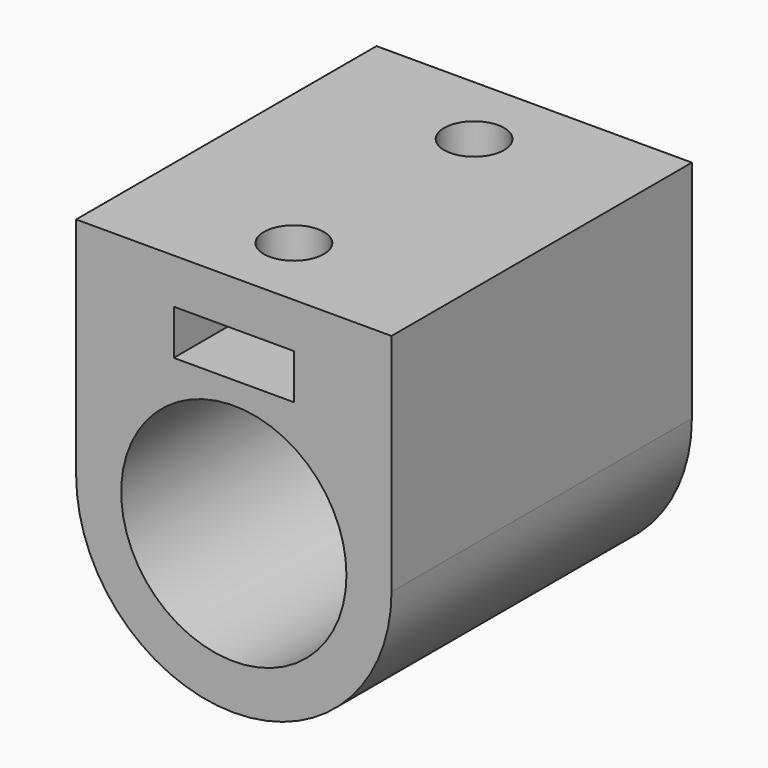
from build123d import *

# Parameters (mm, degrees)
F1_DEPTH        = 25
F2_R            = 2
F3_DEPTH        = 6
F4_W            = 8
F4_H            = 3
F5_DEPTH        = 8
F5_COPIES_COUNT = 2
F5_COPIES_PITCH = 17


# Not quite as in the source:
# - a pattern or mirror of a feature is missing from the dataset's text; its kind, count and spacing are read off the source's solid


with BuildPart() as f1:
    # F0 (on Front) → F1 (new body)
    with BuildSketch(Plane.XZ):
        with BuildLine():
            ThreePointArc((-10.5, 0), (0, 10.5), (10.5, 0))
            Line((10.5, 0), (10.5, 15))
            Line((10.5, 15), (-10.5, 15))
            Line((-10.5, 15), (-10.5, 0))
        make_face()
        with BuildLine():
            Line((10.5, 0), (7.5, 0))
            ThreePointArc((7.5, 0), (0, -7.5), (-7.5, 0))
            Line((-7.5, 0), (-10.5, 0))
            ThreePointArc((-10.5, 0), (0, -10.5), (10.5, 0))
        make_face()
        with BuildLine():
            ThreePointArc((-7.5, 0), (0, 7.5), (7.5, 0))
            Line((7.5, 0), (10.5, 0))
            ThreePointArc((10.5, 0), (0, 10.5), (-10.5, 0))
            Line((-10.5, 0), (-7.5, 0))
        make_face()
    extrude(amount=F1_DEPTH)

    # F2 (on face) → F3 (cut)
    with BuildSketch(Plane.XY.offset(15)):
        with Locations((0, -5)):
            Circle(F2_R)
        with Locations((0, -20)):
            Circle(F2_R)
    extrude(amount=-F3_DEPTH, mode=Mode.SUBTRACT)

    # F4 (on face) → F5 (cut)
    with BuildSketch(Plane.XZ.offset(25)):
        with Locations((0, 10.5)):
            Rectangle(F4_W, F4_H)
    f5 = extrude(amount=-F5_DEPTH, mode=Mode.SUBTRACT)

    # F5_copies: F5 ×2
    with Locations(*[(0, i * F5_COPIES_PITCH, 0) for i in range(1, F5_COPIES_COUNT)]):
        add(f5, mode=Mode.SUBTRACT)


solid = f1.part
